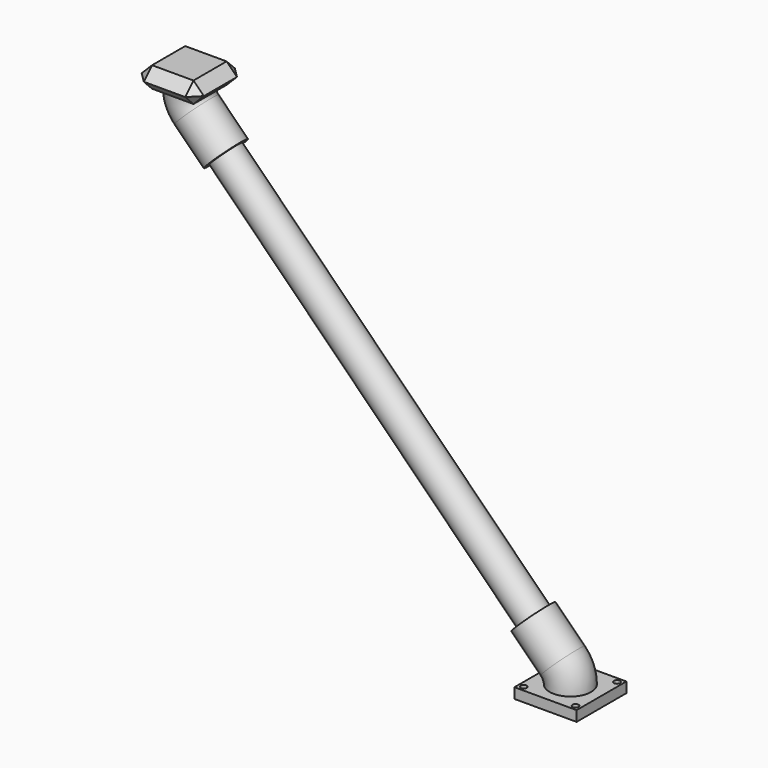
from build123d import *

# Parameters (mm, degrees)
F0_W      = 30
F0_H      = 30
F0_R      = 10
F0_R_2    = 7.5
F1_DEPTH  = 5
F2_ANGLE  = 45
F4_DEPTH  = 20
F3_R      = 7.5
F5_DEPTH  = 250
F6_R      = 10
F6_R_2    = 7.5
F7_ANGLE  = 45
F8_DEPTH  = 20
F9_W      = 30
F9_H      = 30
F9_R      = 10
F10_DEPTH = 10
F11_SIZE  = 4.99999


# Not quite as in the source:
# - a fillet or chamfer is up to 0.001 mm smaller than in the source, because OpenCascade refuses the exact size


with BuildPart() as f1:
    # F0 (on Top) → F1 (new body)
    with BuildSketch(Plane.XY):
        Rectangle(F0_W, F0_H)
        with BuildLine():
            Line((11, -12.5), (-11, -12.5))
            ThreePointArc((-11, -12.5), (-13.5606601718, -13.5606601718), (-12.5, -11))
            Line((-12.5, -11), (-12.5, 11))
            ThreePointArc((-12.5, 11), (-13.5606601718, 13.5606601718), (-11, 12.5))
            Line((-11, 12.5), (11, 12.5))
            ThreePointArc((11, 12.5), (12.5, 14), (14, 12.5))
            ThreePointArc((14, 12.5), (13.5606601718, 11.4393398282), (12.5, 11))
            Line((12.5, 11), (12.5, -11))
            ThreePointArc((12.5, -11), (13.5606601718, -11.4393398282), (14, -12.5))
            ThreePointArc((14, -12.5), (12.5, -14), (11, -12.5))
        make_face(mode=Mode.SUBTRACT)
        with BuildLine():
            ThreePointArc((-12.5, -11), (-11.4393398282, -11.4393398282), (-11, -12.5))
            Line((-11, -12.5), (11, -12.5))
            ThreePointArc((11, -12.5), (11.4393398282, -11.4393398282), (12.5, -11))
            Line((12.5, -11), (12.5, 11))
            ThreePointArc((12.5, 11), (11.4393398282, 11.4393398282), (11, 12.5))
            Line((11, 12.5), (-11, 12.5))
            ThreePointArc((-11, 12.5), (-11.4393398282, 11.4393398282), (-12.5, 11))
            Line((-12.5, 11), (-12.5, -11))
        make_face()
        Circle(F0_R, mode=Mode.SUBTRACT)
        Circle(F0_R)
        Circle(F0_R_2, mode=Mode.SUBTRACT)
        Circle(F0_R_2)
    extrude(amount=-F1_DEPTH)

    # F0 (on Top) → F2 (revolve)
    with BuildSketch(Plane.XY):
        Circle(F0_R)
        Circle(F0_R_2, mode=Mode.SUBTRACT)
    revolve(axis=Axis((-12.5, 0, 0), (0, -1, 0)), revolution_arc=F2_ANGLE)

    # F4 (add): a face of the model
    f4_faces = [f1.faces().sort_by_distance(p)[0] for p in [
        (-10.532233047, 0, 1.967766953),
    ]]
    extrude(f4_faces, amount=F4_DEPTH)


with BuildPart() as f5:
    # F3 (on face) → F5 (new body)
    with BuildSketch(Plane(origin=(-6.25, 0, 6.25), x_dir=(0.7071067812, 0, 0.7071067812), z_dir=(-0.7071067812, 0, 0.7071067812))):
        with Locations((3.6611652352, 0)):
            Circle(F3_R)
    extrude(amount=F5_DEPTH)


with BuildPart() as f7:
    # F6 (on face) → F7 (revolve)
    with BuildSketch(Plane(origin=(-183.0266952966, 0, 183.0266952966), x_dir=(0.7071067812, 0, 0.7071067812), z_dir=(-0.7071067812, 0, 0.7071067812))):
        with Locations((3.6611652352, 0)):
            Circle(F6_R)
        with Locations((3.6611652352, 0)):
            Circle(F6_R_2, mode=Mode.SUBTRACT)
        with Locations((3.6611652352, 0)):
            Circle(F6_R_2)
    revolve(axis=Axis((-171.9525791576, -0.2738032596, 194.1008114357), (0, 1, 0)), revolution_arc=F7_ANGLE)

    # F6 (on face) → F8 (join)
    with BuildSketch(Plane(origin=(-183.0266952966, 0, 183.0266952966), x_dir=(0.7071067812, 0, 0.7071067812), z_dir=(-0.7071067812, 0, 0.7071067812))):
        with Locations((3.6611652352, 0)):
            Circle(F6_R)
        with Locations((3.6611652352, 0)):
            Circle(F6_R_2, mode=Mode.SUBTRACT)
    extrude(amount=-F8_DEPTH)

    # F9 (on face) → F10 (join)
    with BuildSketch(Plane.XY.offset(194.1008114357)):
        with Locations((-183.9525791576, 0)):
            Rectangle(F9_W, F9_H)
        with Locations((-183.9525791576, 0)):
            Circle(F9_R, mode=Mode.SUBTRACT)
        with Locations((-183.9525791576, 0)):
            Circle(F9_R)
    extrude(amount=F10_DEPTH)

    # F11 (size 5 in the source; OpenCascade refuses exactly that, so slightly less here)
    f11_edges = [f7.edges().sort_by_distance(p)[0] for p in [
        (-198.952579, 15, 199.100811),
        (-198.952579, -15, 199.100811),
        (-198.952579, 0, 194.100811),
        (-198.952579, 0, 204.100811),
        (-168.952579, 15, 199.100811),
        (-183.952579, 15, 194.100811),
        (-183.952579, 15, 204.100811),
        (-168.952579, -15, 199.100811),
        (-168.952579, 0, 194.100811),
        (-168.952579, 0, 204.100811),
        (-183.952579, -15, 194.100811),
        (-183.952579, -15, 204.100811),
    ]]
    chamfer(f11_edges, length=F11_SIZE)


solid = Compound([f1.part, f5.part, f7.part])
